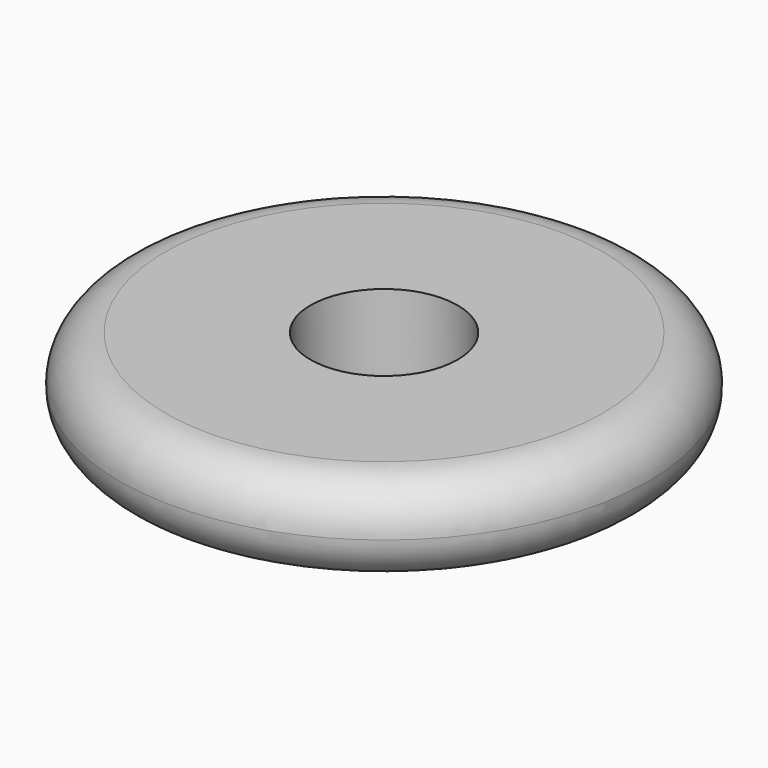
from build123d import *

# Parameters (mm, degrees)
F0_R     = 11.65
F1_DEPTH = 4
F2_R     = 1.99999
F3_R     = 3.25
F4_DEPTH = 25


# Not quite as in the source:
# - a fillet or chamfer is up to 0.001 mm smaller than in the source, because OpenCascade refuses the exact size


with BuildPart() as f1:
    # F0 (on Top) → F1 (new body)
    with BuildSketch(Plane.XY):
        Circle(F0_R)
    extrude(amount=F1_DEPTH)

    # F2 (radius 2 in the source; OpenCascade refuses exactly that, so slightly less here)
    f2_edges = [f1.edges().sort_by_distance(p)[0] for p in [
        (-11.65, 0, 4),
        (-11.65, 0, 0),
    ]]
    fillet(f2_edges, radius=F2_R)

    # F3 (on face) → F4 (cut)
    with BuildSketch(Plane.XY.offset(4)):
        Circle(F3_R)
    extrude(amount=-F4_DEPTH, mode=Mode.SUBTRACT)


solid = f1.part
